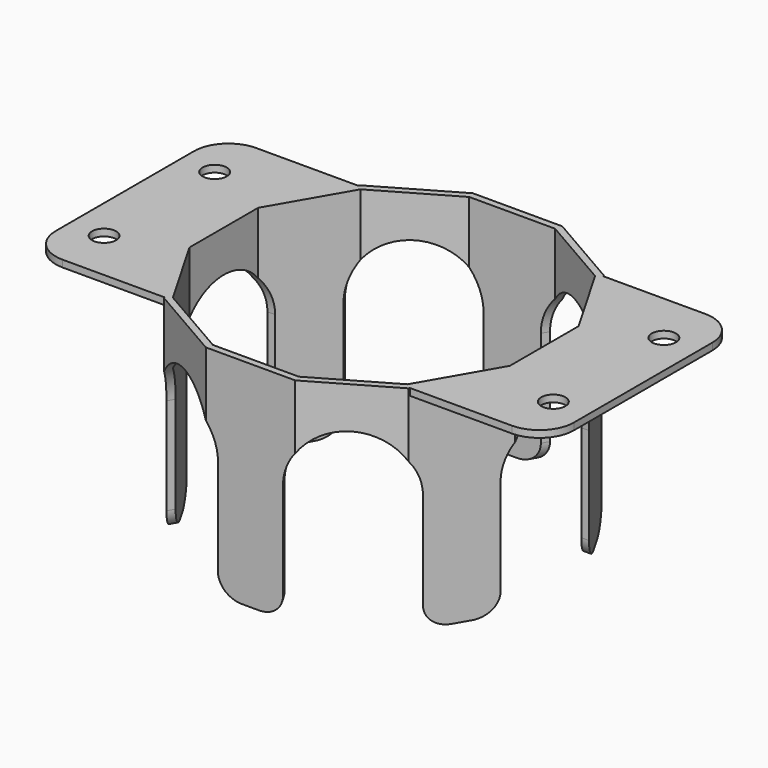
from build123d import *

# Parameters (mm, degrees)
F0_W             = 75
F0_H             = 35
F1_DEPTH         = 1
F3_DEPTH         = 30
F5_DEPTH         = 35
F6_R             = 5
F7_R             = 1.75
F8_DEPTH         = 25
F9_DEPTH         = 1
F10_DEPTH        = 65.4
F13_DEPTH        = 35.6
F13_COPIES_COUNT = 6
F14_T1_DEPTH     = 16.1153550717
F14_T3_DEPTH     = 16.1153550717
F14_T5_DEPTH     = 16.1153550717
F14_T7_DEPTH     = 16.1153550717
F14_T9_DEPTH     = 16.1153550717
F14_T11_DEPTH    = 16.1153550717
F14_T13_DEPTH    = 16.1153550717
F14_T15_DEPTH    = 16.1153550717
F14_T17_DEPTH    = 16.1153550717
F14_T19_DEPTH    = 16.1153550717


# Not quite as in the source:
# - a fillet or chamfer that OpenCascade refuses, or shapes differently, is made with other operations: its cross-section is extruded or revolved along the edge and cut away or added
# - a pattern or mirror of a feature is missing from the dataset's text; its kind, count and spacing are read off the source's solid


with BuildPart() as f1:
    # F0 (on Top) → F1 (new body)
    with BuildSketch(Plane.XY):
        Rectangle(F0_W, F0_H)
    extrude(amount=F1_DEPTH)

    # F2 (on Top) → F3 (join)
    with BuildSketch(Plane.XY):
        Polygon((24.1481456572, 6.4704761276), (17.6776695297, 17.6776695297), (6.4704761276, 24.1481456572), (-6.4704761276, 24.1481456572), (-17.6776695297, 17.6776695297), (-24.1481456572, 6.4704761276), (-24.1481456572, -6.4704761276), (-17.6776695297, -17.6776695297), (-6.4704761276, -24.1481456572), (6.4704761276, -24.1481456572), (17.6776695297, -17.6776695297), (24.1481456572, -6.4704761276), align=None)
    extrude(amount=-F3_DEPTH)

    # F4 (on face) → F5 (cut)
    with BuildSketch(Plane(origin=(0, 0, -30), x_dir=(1, 0, 0), z_dir=(0, 0, -1))):
        Polygon((6.2116570825, -23.1822198309), (16.9705627485, -16.9705627485), (23.1822198309, -6.2116570825), (23.1822198309, 6.2116570825), (16.9705627485, 16.9705627485), (6.2116570825, 23.1822198309), (-6.2116570825, 23.1822198309), (-16.9705627485, 16.9705627485), (-23.1822198309, 6.2116570825), (-23.1822198309, -6.2116570825), (-16.9705627485, -16.9705627485), (-6.2116570825, -23.1822198309), align=None)
    extrude(amount=-F5_DEPTH, mode=Mode.SUBTRACT)

    # F6
    f6_edges = [f1.edges().sort_by_distance(p)[0] for p in [
        (37.5, -17.5, 0.5),
        (37.5, 17.5, 0.5),
        (-37.5, -17.5, 0.5),
        (-37.5, 17.5, 0.5),
    ]]
    fillet(f6_edges, radius=F6_R)

    # F7 (on Top) → F8 (cut)
    with BuildSketch(Plane.XY):
        with Locations((-32.5, 10)):
            Circle(F7_R)
        with Locations((-32.5, -10)):
            Circle(F7_R)
        with Locations((32.5, -10)):
            Circle(F7_R)
        with Locations((32.5, 10)):
            Circle(F7_R)
    extrude(amount=F8_DEPTH, mode=Mode.SUBTRACT)

    # F2 (on Top) → F9 (join)
    with BuildSketch(Plane.XY):
        Polygon((24.1481456572, 6.4704761276), (17.6776695297, 17.6776695297), (6.4704761276, 24.1481456572), (-6.4704761276, 24.1481456572), (-17.6776695297, 17.6776695297), (-24.1481456572, 6.4704761276), (-24.1481456572, -6.4704761276), (-17.6776695297, -17.6776695297), (-6.4704761276, -24.1481456572), (6.4704761276, -24.1481456572), (17.6776695297, -17.6776695297), (24.1481456572, -6.4704761276), align=None)
    extrude(amount=F9_DEPTH)

    # F4 (on face) → F10 (cut)
    with BuildSketch(Plane(origin=(0, 0, -30), x_dir=(1, 0, 0), z_dir=(0, 0, -1))):
        Polygon((6.2116570825, -23.1822198309), (16.9705627485, -16.9705627485), (23.1822198309, -6.2116570825), (23.1822198309, 6.2116570825), (16.9705627485, 16.9705627485), (6.2116570825, 23.1822198309), (-6.2116570825, 23.1822198309), (-16.9705627485, 16.9705627485), (-23.1822198309, 6.2116570825), (-23.1822198309, -6.2116570825), (-16.9705627485, -16.9705627485), (-6.2116570825, -23.1822198309), align=None)
    extrude(amount=-F10_DEPTH, mode=Mode.SUBTRACT)

    # F12 (on Right) → F13 (cut)
    with BuildSketch(Plane.YZ):
        with BuildLine():
            ThreePointArc((-8, -13), (0, -21), (8, -13))
            ThreePointArc((8, -13), (0, -5), (-8, -13))
        make_face()
        with BuildLine():
            Line((8, -37.0977148414), (8, -13))
            ThreePointArc((8, -13), (0, -21), (-8, -13))
            Line((-8, -13), (-8, -36.2910553813))
            Line((-8, -36.2910553813), (8, -37.0977148414))
        make_face()
    f13 = extrude(amount=F13_DEPTH, mode=Mode.SUBTRACT)

    # F13_copies: F13 ×6 about axis
    f13_copies_axis = Axis((0, 0, 0), (0, 0, 1))
    for i in range(1, F13_COPIES_COUNT):
        add(f13.rotate(f13_copies_axis, i * 360 / F13_COPIES_COUNT), mode=Mode.SUBTRACT)

    # F14: fillet of radius 3 on 12 edges, made by hand

    # F14_s2 → F14_t1 (cut)
    with BuildSketch(Plane.YZ.offset(14.6497195661)):
        with BuildLine():
            ThreePointArc((-11, -30), (-8.8786796564, -29.1213203436), (-8, -27))
            Line((-8, -27), (-8, -30))
            Line((-8, -30), (-11, -30))
        make_face()
        with BuildLine():
            ThreePointArc((8, -27), (8.8786796564, -29.1213203436), (11, -30))
            Line((11, -30), (8, -30))
            Line((8, -30), (8, -27))
        make_face()
    extrude(amount=F14_T1_DEPTH, mode=Mode.SUBTRACT)

    # F14_s4 → F14_t3 (cut)
    with BuildSketch(Plane.YZ.offset(-30.7650746377)):
        with BuildLine():
            ThreePointArc((-8, -27), (-8.8786796564, -29.1213203436), (-11, -30))
            Line((-11, -30), (-8, -30))
            Line((-8, -30), (-8, -27))
        make_face()
        with BuildLine():
            ThreePointArc((8, -27), (8.8786796564, -29.1213203436), (11, -30))
            Line((11, -30), (8, -30))
            Line((8, -30), (8, -27))
        make_face()
    extrude(amount=F14_T3_DEPTH, mode=Mode.SUBTRACT)

    # F14_s6 → F14_t5 (cut)
    with BuildSketch(Plane(origin=(-15.3825373189, -26.6433361856, 0), x_dir=(0, 0, 1), z_dir=(0.5, 0.8660254038, 0))):
        with BuildLine():
            ThreePointArc((-30, -11), (-29.1213203436, -8.8786796564), (-27, -8))
            Line((-27, -8), (-30, -8))
            Line((-30, -8), (-30, -11))
        make_face()
    extrude(amount=F14_T5_DEPTH, mode=Mode.SUBTRACT)

    # F14_s8 → F14_t7 (cut)
    with BuildSketch(Plane(origin=(-7.324859783, 12.6870293026, 0), x_dir=(0, 0, 1), z_dir=(-0.5, 0.8660254038, 0))):
        with BuildLine():
            ThreePointArc((-30, -11), (-29.1213203436, -8.8786796564), (-27, -8))
            Line((-27, -8), (-30, -8))
            Line((-30, -8), (-30, -11))
        make_face()
    extrude(amount=F14_T7_DEPTH, mode=Mode.SUBTRACT)

    # F14_s10 → F14_t9 (cut)
    with BuildSketch(Plane(origin=(-7.324859783, -12.6870293026, 0), x_dir=(0, 0, 1), z_dir=(-0.5, -0.8660254038, 0))):
        with BuildLine():
            ThreePointArc((-27, -8), (-29.1213203436, -8.8786796564), (-30, -11))
            Line((-30, -11), (-30, -8))
            Line((-30, -8), (-27, -8))
        make_face()
    extrude(amount=F14_T9_DEPTH, mode=Mode.SUBTRACT)

    # F14_s12 → F14_t11 (cut)
    with BuildSketch(Plane(origin=(7.324859783, 12.6870293026, 0), x_dir=(0, 0, 1), z_dir=(0.5, 0.8660254038, 0))):
        with BuildLine():
            ThreePointArc((-27, -8), (-29.1213203436, -8.8786796564), (-30, -11))
            Line((-30, -11), (-30, -8))
            Line((-30, -8), (-27, -8))
        make_face()
    extrude(amount=F14_T11_DEPTH, mode=Mode.SUBTRACT)

    # F14_s14 → F14_t13 (cut)
    with BuildSketch(Plane(origin=(-15.3825373189, 26.6433361856, 0), x_dir=(0, 0, 1), z_dir=(0.5, -0.8660254038, 0))):
        with BuildLine():
            ThreePointArc((-30, -11), (-29.1213203436, -8.8786796564), (-27, -8))
            Line((-27, -8), (-30, -8))
            Line((-30, -8), (-30, -11))
        make_face()
    extrude(amount=F14_T13_DEPTH, mode=Mode.SUBTRACT)

    # F14_s16 → F14_t15 (cut)
    with BuildSketch(Plane(origin=(15.3825373189, -26.6433361856, 0), x_dir=(0, 0, 1), z_dir=(-0.5, 0.8660254038, 0))):
        with BuildLine():
            ThreePointArc((-30, -11), (-29.1213203436, -8.8786796564), (-27, -8))
            Line((-27, -8), (-30, -8))
            Line((-30, -8), (-30, -11))
        make_face()
    extrude(amount=F14_T15_DEPTH, mode=Mode.SUBTRACT)

    # F14_s18 → F14_t17 (cut)
    with BuildSketch(Plane(origin=(15.3825373189, 26.6433361856, 0), x_dir=(0, 0, 1), z_dir=(-0.5, -0.8660254038, 0))):
        with BuildLine():
            ThreePointArc((-30, -11), (-29.1213203436, -8.8786796564), (-27, -8))
            Line((-27, -8), (-30, -8))
            Line((-30, -8), (-30, -11))
        make_face()
    extrude(amount=F14_T17_DEPTH, mode=Mode.SUBTRACT)

    # F14_s20 → F14_t19 (cut)
    with BuildSketch(Plane(origin=(7.324859783, -12.6870293026, 0), x_dir=(0, 0, 1), z_dir=(0.5, -0.8660254038, 0))):
        with BuildLine():
            ThreePointArc((-27, -8), (-29.1213203436, -8.8786796564), (-30, -11))
            Line((-30, -11), (-30, -8))
            Line((-30, -8), (-27, -8))
        make_face()
    extrude(amount=F14_T19_DEPTH, mode=Mode.SUBTRACT)


solid = f1.part
